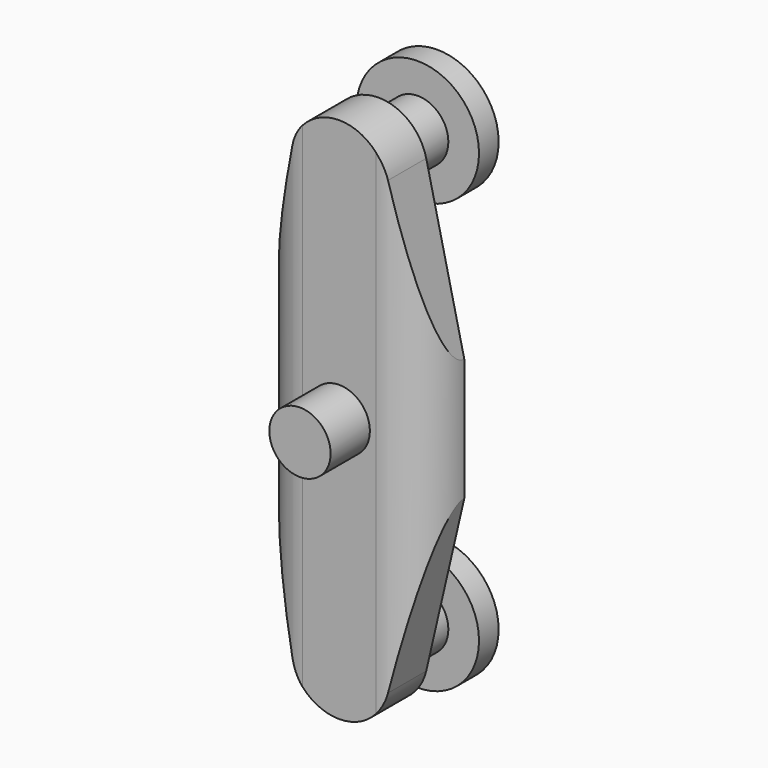
from build123d import *

# Parameters (mm, degrees)
F0_R     = 6.35
F1_DEPTH = 2.54
F2_R     = 3.175
F3_DEPTH = 5.08
F4_R     = 3.175
F4_W     = 17.78
F4_H     = 12.7
F5_DEPTH = 5.08
F7_R     = 5.07999
F8_R     = 3.175
F9_DEPTH = 5.08


# Not quite as in the source:
# - a fillet or chamfer is up to 0.001 mm smaller than in the source, because OpenCascade refuses the exact size


with BuildPart() as f1:
    # F0 (on Front) → F1 (new body)
    with BuildSketch(Plane.XZ):
        with Locations((0, 22.225)):
            Circle(F0_R)
    extrude(amount=F1_DEPTH)

    # F2 (on face) → F3 (join)
    with BuildSketch(Plane.XZ.offset(2.54)):
        with Locations((0, 22.225)):
            Circle(F2_R)
    extrude(amount=F3_DEPTH)

    # F4 (on face) → F5 (join)
    with BuildSketch(Plane.XZ.offset(7.62)):
        with BuildLine():
            ThreePointArc((4.9490759915, 23.3708825552), (5.0471628682, 22.8016688665), (5.08, 22.225))
            ThreePointArc((5.08, 22.225), (-0.5766688665, 17.1778371318), (-4.9490759915, 23.3708825552))
            Line((-4.9490759915, 23.3708825552), (-8.89, 6.35))
            Line((-8.89, 6.35), (8.89, 6.35))
            Line((8.89, 6.35), (4.9490759915, 23.3708825552))
        make_face()
        with BuildLine():
            ThreePointArc((-4.9490759915, 23.3708825552), (-0.5766688665, 17.1778371318), (5.08, 22.225))
            ThreePointArc((5.08, 22.225), (5.0471628682, 22.8016688665), (4.9490759915, 23.3708825552))
            ThreePointArc((4.9490759915, 23.3708825552), (0, 27.305), (-4.9490759915, 23.3708825552))
        make_face()
        with Locations((0, 22.225)):
            Circle(F4_R, mode=Mode.SUBTRACT)
        with Locations((0, 22.225)):
            Circle(F4_R)
        Rectangle(F4_W, F4_H)
    extrude(amount=F5_DEPTH)

    # F6: F1 across plane


with BuildPart() as f1_1:
    add(f1.part)
    add(f1.part.mirror(Plane.XY))

    # F7 (radius 5.08 in the source; OpenCascade refuses exactly that, so slightly less here)
    f7_edges = [f1_1.edges().sort_by_distance(p)[0] for p in [
        (-8.89, -12.7, 0),
        (8.89, -12.7, 0),
    ]]
    fillet(f7_edges, radius=F7_R)

    # F8 (on face) → F9 (join)
    with BuildSketch(Plane.XZ.offset(12.7)):
        Circle(F8_R)
    extrude(amount=F9_DEPTH)


solid = f1_1.part
